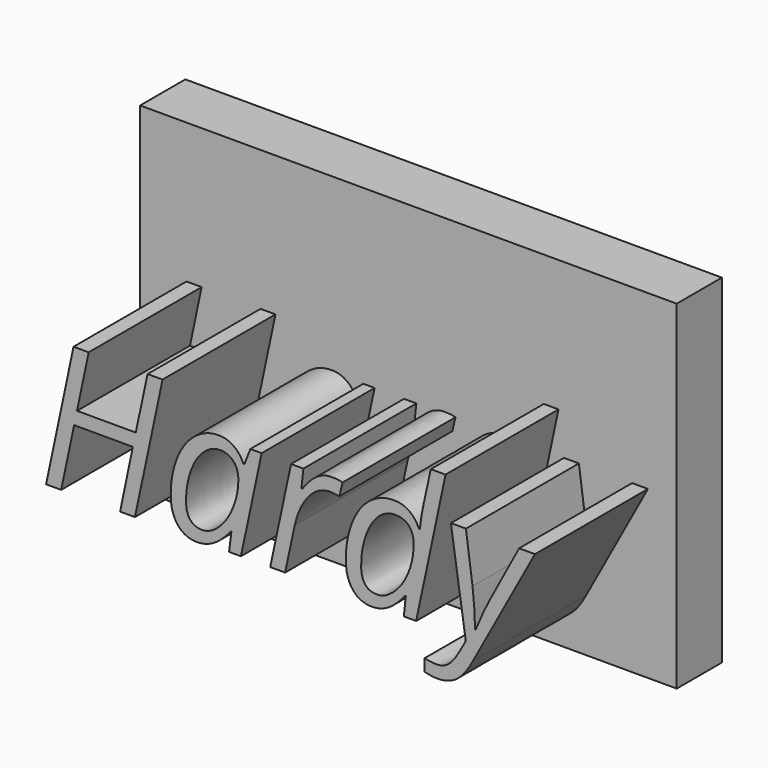
from build123d import *

# Parameters (mm, degrees)
F0_W         = 24.13
F0_H         = 15.24
F1_DEPTH     = 2.54
F2_TEXT_SIZE = 8.1935483871
F3_DEPTH     = 6.35


# Not quite as in the source:
# - Text() gives the source's letters only with a copy of the font that has no kerning and outlines rounded to 1/6400 em; it was checked with that copy


with BuildPart() as f1:
    # F0 (on Front) → F1 (new body)
    with BuildSketch(Plane.XZ):
        Rectangle(F0_W, F0_H)
    extrude(amount=F1_DEPTH)

    # F2 (on face) → F3 (join)
    with BuildSketch(Plane.XZ.offset(2.54)):
        with Locations((-11.559481787, -4.5202797043)):
            Text('Hardy', F2_TEXT_SIZE, font='Open Sans', font_style=FontStyle.ITALIC, text_align=(TextAlign.LEFT, TextAlign.BOTTOM))
    extrude(amount=F3_DEPTH)


solid = f1.part
